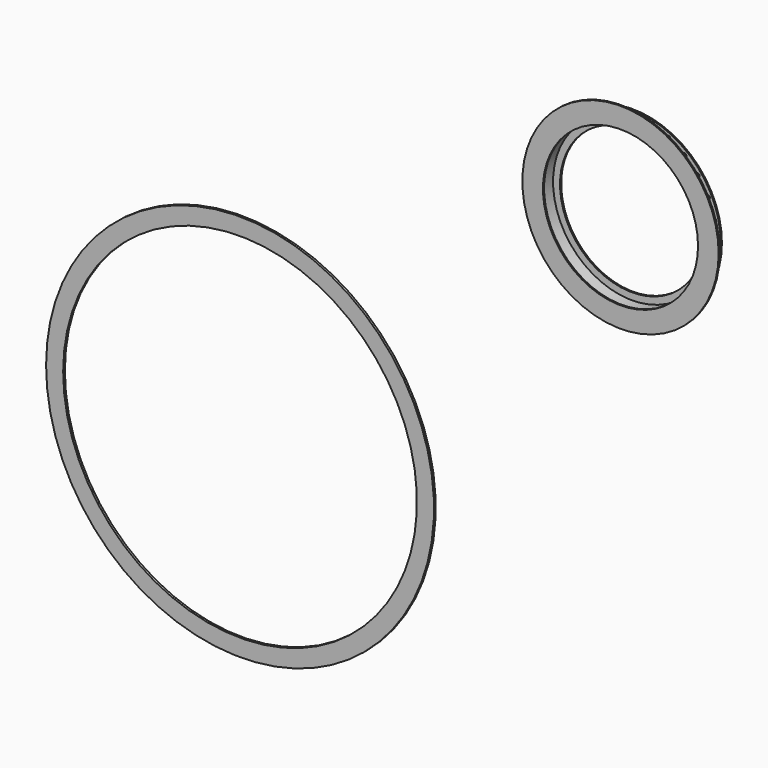
from build123d import *

# Parameters (mm, degrees)
F0_R             = 625
F0_R_2           = 505
F1_DEPTH         = 10
F2_R             = 560
F2_R_2           = 554
F3_DEPTH         = 90
F4_R             = 690
F4_R_2           = 545
F5_DEPTH         = 10
F7_R             = 1363.5
F7_R_2           = 1243.5
F8_DEPTH         = 15
F14_R            = 12
F15_DEPTH        = 10
F15_COPIES_COUNT = 28


# Not quite as in the source:
# - a pattern or mirror of a feature is missing from the dataset's text; its kind, count and spacing are read off the source's solid
# - the program builds the solid bodies; features that only make, move or delete a surface that nothing else refers to are left out


with BuildPart() as f1:
    # F0 (on Front) → F1 (new body)
    with BuildSketch(Plane.XZ):
        Circle(F0_R)
        Circle(F0_R_2, mode=Mode.SUBTRACT)
    extrude(amount=-F1_DEPTH)

    # F2 (on face) → F3 (join)
    with BuildSketch(Plane.XZ):
        Circle(F2_R)
        Circle(F2_R_2, mode=Mode.SUBTRACT)
    extrude(amount=F3_DEPTH)

    # F4 (on face) → F5 (join)
    with BuildSketch(Plane.XZ.offset(90)):
        Circle(F4_R)
        Circle(F4_R_2, mode=Mode.SUBTRACT)
    extrude(amount=F5_DEPTH)

    # F14 (on face) → F15 (cut, through all)
    with BuildSketch(Plane(origin=(0, 10, 0), x_dir=(-1, 0, 0), z_dir=(0, 1, 0))):
        with Locations((595, 0)):
            Circle(F14_R)
    f15 = extrude(amount=-F15_DEPTH, mode=Mode.SUBTRACT)

    # F15_copies: F15 ×28 about axis
    f15_copies_axis = Axis((0, 0, 0), (0, 1, 0))
    for i in range(1, F15_COPIES_COUNT):
        add(f15.rotate(f15_copies_axis, i * 360 / F15_COPIES_COUNT), mode=Mode.SUBTRACT)


with BuildPart() as f8:
    # F7 (on offset) → F8 (new body)
    with BuildSketch(Plane(origin=(0, -3443, 0), x_dir=(-1, 0, 0), z_dir=(0, 1, 0))):
        Circle(F7_R)
        Circle(F7_R_2, mode=Mode.SUBTRACT)
    extrude(amount=F8_DEPTH)


solid = Compound([f1.part, f8.part])
